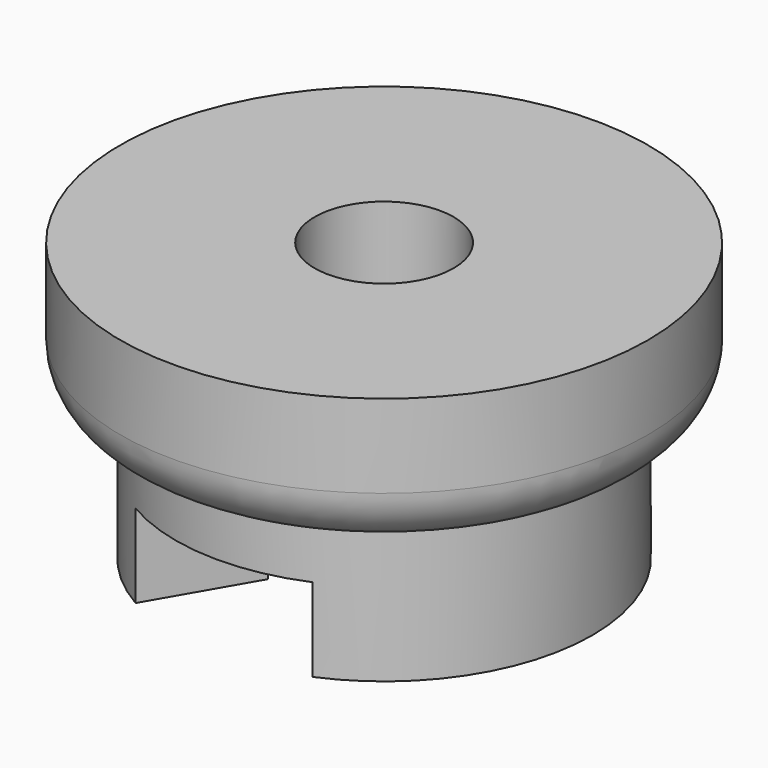
from build123d import *

# Parameters (mm, degrees)
F2_R     = 1.99999
F4_DEPTH = 3


# Not quite as in the source:
# - a fillet or chamfer is up to 0.001 mm smaller than in the source, because OpenCascade refuses the exact size
# - a feature names something its author has since deleted; it is built from what else it names


with BuildPart() as f1:
    # F0 (on Front) → F1 (revolve)
    with BuildSketch(Plane.XZ):
        Polygon((2.5, 2), (3.5, 2), (3.5, 0), (7.5, 0), (7.5, 5), (9.5, 5), (9.5, 10), (2.5, 10), align=None)
    revolve(axis=Axis((0, 0, 8.8058942929), (0, 0, 1)))

    # F2 (radius 2 in the source; OpenCascade refuses exactly that, so slightly less here)
    f2_edges = [f1.edges().sort_by_distance(p)[0] for p in [
        (-9.5, 0, 5),
    ]]
    fillet(f2_edges, radius=F2_R)

    # F3 (on face) → F4 (cut)
    with BuildSketch(Plane(origin=(0, 0, 0), x_dir=(1, 0, 0), z_dir=(0, 0, -1))):
        with BuildLine():
            ThreePointArc((-1.75, 3.0310889132), (0.8206712512, 3.402425414), (2.9393876913, 1.9))
            Line((2.9393876913, 1.9), (2.9393876913, 6.9))
            ThreePointArc((2.9393876913, 6.9), (-0.4530350492, 7.486304779), (-3.75, 6.4951905284))
            Line((-3.75, 6.4951905284), (-1.75, 3.0310889132))
        make_face()
    extrude(amount=-F4_DEPTH, mode=Mode.SUBTRACT)


solid = f1.part
